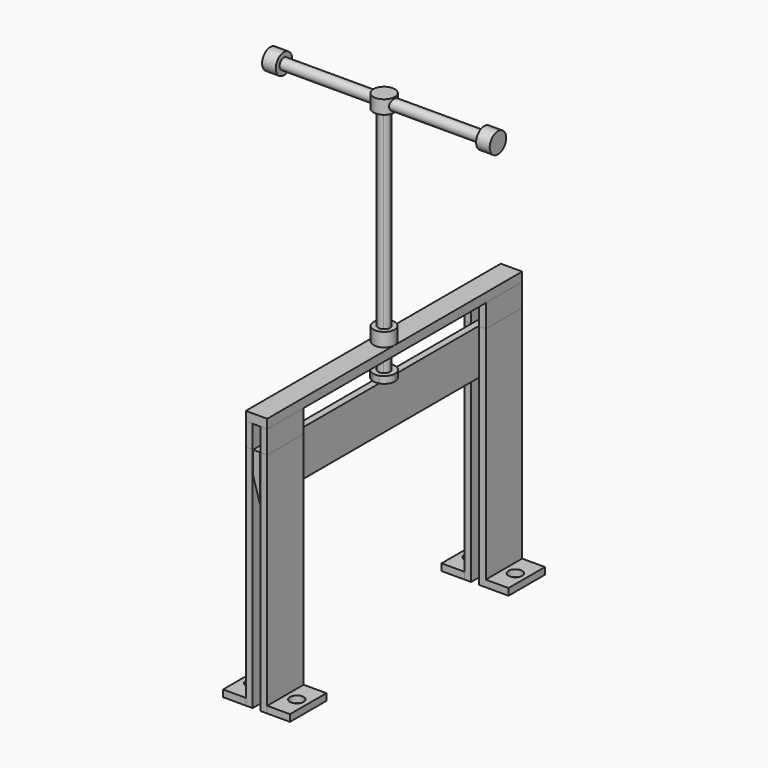
from build123d import *

# Parameters (mm, degrees)
F0_W      = 1.5
F0_H      = 70
F1_DEPTH  = 10
F3_DEPTH  = 70.001
F4_W      = 1.5
F4_H      = 10
F5_DEPTH  = 50
F6_DEPTH  = 5
F7_W      = 4.7004564702
F7_H      = 70.0002348423
F8_DEPTH  = 2
F11_DEPTH = 55
F9_R      = 2.3144907663
F12_DEPTH = 3
F13_R     = 2.3453015316
F13_R_2   = 1.3011317458
F14_DEPTH = 3
F15_R     = 1.186628288
F16_DEPTH = 25
F17_R     = 2.2512446739
F17_R_2   = 1.186628288
F18_DEPTH = 3
F19_DEPTH = 25
F20_R     = 2.2550084993
F20_R_2   = 1.186628288
F21_DEPTH = 3
F22_W     = 5
F22_H     = 10
F23_DEPTH = 1.5
F24_W     = 5
F24_H     = 10
F25_DEPTH = 1.5
F24_W_2   = 4.9965837158
F27_R     = 1.5
F28_DEPTH = 1.501
F26_R     = 1.5
F29_DEPTH = 1.501
F31_R     = 1.5
F32_DEPTH = 1.501
F30_R     = 1.5
F33_DEPTH = 1.501
F35_DEPTH = 1.5


# Not quite as in the source:
# - the program builds the solid bodies; features that only make, move or delete a surface that nothing else refers to are left out


with BuildPart() as f1:
    # F0 (on Top) → F1 (new body)
    with BuildSketch(Plane.XY):
        with Locations((-0.0246972009, 0)):
            Rectangle(F0_W, F0_H)
    extrude(amount=-F1_DEPTH)

    # F2 (on face) → F3 (cut, through all)
    with BuildSketch(Plane.XZ.offset(35)):
        Polygon((0.7253027991, -10), (-0.7746972009, -5), (-0.7746972009, -10), align=None)
    extrude(amount=-F3_DEPTH, mode=Mode.SUBTRACT)


with BuildPart() as f5:
    # F4 (on face) → F5 (new body)
    with BuildSketch(Plane.XY):
        with Locations((1.5753027991, 30)):
            Rectangle(F4_W, F4_H)
    extrude(amount=-F5_DEPTH)

    # F24 (on face) → F25 (join)
    with BuildSketch(Plane(origin=(0, 0, -50), x_dir=(1, 0, 0), z_dir=(0, 0, -1))):
        with Locations((4.8253027991, -30)):
            Rectangle(F24_W, F24_H)
    extrude(amount=-F25_DEPTH)

    # F26 (on face) → F29 (cut, through all)
    with BuildSketch(Plane.XY.offset(-48.5)):
        with Locations((4.8253027991, 30)):
            Circle(F26_R)
    extrude(amount=-F29_DEPTH, mode=Mode.SUBTRACT)


with BuildPart() as f5b:
    # F4 (on face) → F5, piece 2 (new body)
    with BuildSketch(Plane.XY):
        with Locations((-1.6246972009, 30)):
            Rectangle(F4_W, F4_H)
    extrude(amount=-F5_DEPTH)


with BuildPart() as f5c:
    # F4 (on face) → F5, piece 3 (new body)
    with BuildSketch(Plane.XY):
        with Locations((-1.6246972009, -30)):
            Rectangle(F4_W, F4_H)
    extrude(amount=-F5_DEPTH)


with BuildPart() as f5d:
    # F4 (on face) → F5, piece 4 (new body)
    with BuildSketch(Plane.XY):
        with Locations((1.5753027991, -30)):
            Rectangle(F4_W, F4_H)
    extrude(amount=-F5_DEPTH)


with BuildPart() as f6:
    # F4 (on face) → F6 (new body)
    with BuildSketch(Plane.XY):
        with Locations((-1.6246972009, 30)):
            Rectangle(F4_W, F4_H)
    extrude(amount=F6_DEPTH)


with BuildPart() as f6b:
    # F4 (on face) → F6, piece 2 (new body)
    with BuildSketch(Plane.XY):
        with Locations((1.5753027991, 30)):
            Rectangle(F4_W, F4_H)
    extrude(amount=F6_DEPTH)


with BuildPart() as f6c:
    # F4 (on face) → F6, piece 3 (new body)
    with BuildSketch(Plane.XY):
        with Locations((-1.6246972009, -30)):
            Rectangle(F4_W, F4_H)
    extrude(amount=F6_DEPTH)


with BuildPart() as f6d:
    # F4 (on face) → F6, piece 4 (new body)
    with BuildSketch(Plane.XY):
        with Locations((1.5753027991, -30)):
            Rectangle(F4_W, F4_H)
    extrude(amount=F6_DEPTH)


with BuildPart() as f8:
    # F7 (on face) → F8 (new body)
    with BuildSketch(Plane.XY.offset(5)):
        with Locations((-0.0244689658, -0.0001174212)):
            Rectangle(F7_W, F7_H)
    extrude(amount=F8_DEPTH)


with BuildPart() as f11:
    # F10 (on face) → F11 (new body)
    with BuildSketch(Plane.XY):
        with BuildLine():
            Line((-0.7746972009, -1.0453650399), (-0.7746972009, 1.0453650399))
            ThreePointArc((-0.7746972009, 1.0453650399), (-1.3011317458, 0), (-0.7746972009, -1.0453650399))
        make_face()
        with BuildLine():
            ThreePointArc((0.7253027991, -1.0802220464), (1.1481851586, -0.6120577271), (1.3011317458, 0))
            ThreePointArc((1.3011317458, 0), (1.1481851586, 0.6120577271), (0.7253027991, 1.0802220464))
            Line((0.7253027991, 1.0802220464), (0.7253027991, -1.0802220464))
        make_face()
        with BuildLine():
            Line((0.7253027991, -1.0802220464), (0.7253027991, 1.0802220464))
            ThreePointArc((0.7253027991, 1.0802220464), (-0.0302275447, 1.3007805792), (-0.7746972009, 1.0453650399))
            Line((-0.7746972009, 1.0453650399), (-0.7746972009, -1.0453650399))
            ThreePointArc((-0.7746972009, -1.0453650399), (-0.0302275447, -1.3007805792), (0.7253027991, -1.0802220464))
        make_face()
    extrude(amount=F11_DEPTH)

    # F13 (on face) → F14 (join)
    with BuildSketch(Plane.XY.offset(55)):
        Circle(F13_R)
        Circle(F13_R_2, mode=Mode.SUBTRACT)
    extrude(amount=-F14_DEPTH)

    # F15 (on Right) → F16 (join)
    with BuildSketch(Plane.YZ):
        with Locations((0, 53.5126663744)):
            Circle(F15_R)
    extrude(amount=-F16_DEPTH)

    # F17 (on face) → F18 (join)
    with BuildSketch(Plane(origin=(-25, 0, 0), x_dir=(0, -1, 0), z_dir=(-1, 0, 0))):
        with Locations((0, 53.5126663744)):
            Circle(F17_R)
        with Locations((0, 53.5126663744)):
            Circle(F17_R_2, mode=Mode.SUBTRACT)
    extrude(amount=-F18_DEPTH)

    # F15 (on Right) → F19 (join)
    with BuildSketch(Plane.YZ):
        with Locations((0, 53.5126663744)):
            Circle(F15_R)
    extrude(amount=F19_DEPTH)

    # F20 (on face) → F21 (join)
    with BuildSketch(Plane.YZ.offset(25)):
        with Locations((0, 53.5126663744)):
            Circle(F20_R)
        with Locations((0, 53.5126663744)):
            Circle(F20_R_2, mode=Mode.SUBTRACT)
    extrude(amount=-F21_DEPTH)


with BuildPart() as f12:
    # F9 (on face) → F12 (new body)
    with BuildSketch(Plane.XY.offset(7)):
        Circle(F9_R)
    extrude(amount=F12_DEPTH)


with BuildPart() as f23:
    # F22 (on face) → F23 (new body)
    with BuildSketch(Plane(origin=(0, 0, -50), x_dir=(1, 0, 0), z_dir=(0, 0, -1))):
        with Locations((4.8253027991, 30)):
            Rectangle(F22_W, F22_H)
    extrude(amount=-F23_DEPTH)

    # F30 (on face) → F33 (cut, through all)
    with BuildSketch(Plane.XY.offset(-48.5)):
        with Locations((4.8253027991, -30)):
            Circle(F30_R)
    extrude(amount=-F33_DEPTH, mode=Mode.SUBTRACT)


with BuildPart() as f23b:
    # F22 (on face) → F23, piece 2 (new body)
    with BuildSketch(Plane(origin=(0, 0, -50), x_dir=(1, 0, 0), z_dir=(0, 0, -1))):
        with Locations((-4.8746972009, 30)):
            Rectangle(F22_W, F22_H)
    extrude(amount=-F23_DEPTH)

    # F31 (on face) → F32 (cut, through all)
    with BuildSketch(Plane.XY.offset(-48.5)):
        with Locations((-4.8746972009, -30)):
            Circle(F31_R)
    extrude(amount=-F32_DEPTH, mode=Mode.SUBTRACT)


with BuildPart() as f25:
    # F24 (on face) → F25, piece 2 (new body)
    with BuildSketch(Plane(origin=(0, 0, -50), x_dir=(1, 0, 0), z_dir=(0, 0, -1))):
        with Locations((-4.8763835644, -29.9852424113)):
            Rectangle(F24_W_2, F24_H)
    extrude(amount=-F25_DEPTH)

    # F27 (on face) → F28 (cut, through all)
    with BuildSketch(Plane.XY.offset(-48.5)):
        with Locations((-4.8763835644, 29.9852424113)):
            Circle(F27_R)
    extrude(amount=-F28_DEPTH, mode=Mode.SUBTRACT)


with BuildPart() as f35:
    # F34 (on face) → F35 (new body)
    with BuildSketch(Plane.XY):
        with BuildLine():
            Line((-0.7746972009, -2.2538692437), (-0.7746972009, 2.2538692437))
            ThreePointArc((-0.7746972009, 2.2538692437), (-2.383292328, 0), (-0.7746972009, -2.2538692437))
        make_face()
        with BuildLine():
            Line((0.7253027991, -2.2702462797), (0.7253027991, 2.2702462797))
            ThreePointArc((0.7253027991, 2.2702462797), (-0.0260192921, 2.3831502926), (-0.7746972009, 2.2538692437))
            Line((-0.7746972009, 2.2538692437), (-0.7746972009, -2.2538692437))
            ThreePointArc((-0.7746972009, -2.2538692437), (-0.0260192921, -2.3831502926), (0.7253027991, -2.2702462797))
        make_face()
        with BuildLine():
            ThreePointArc((0.7253027991, -2.2702462797), (1.9246676229, -1.4056090716), (2.383292328, 0))
            ThreePointArc((2.383292328, 0), (1.9246676229, 1.4056090716), (0.7253027991, 2.2702462797))
            Line((0.7253027991, 2.2702462797), (0.7253027991, -2.2702462797))
        make_face()
    extrude(amount=F35_DEPTH)


solid = Compound([f1.part, f5.part, f5b.part, f5c.part, f5d.part, f6.part, f6b.part, f6c.part, f6d.part, f8.part, f11.part, f12.part, f23.part, f23b.part, f25.part, f35.part])
